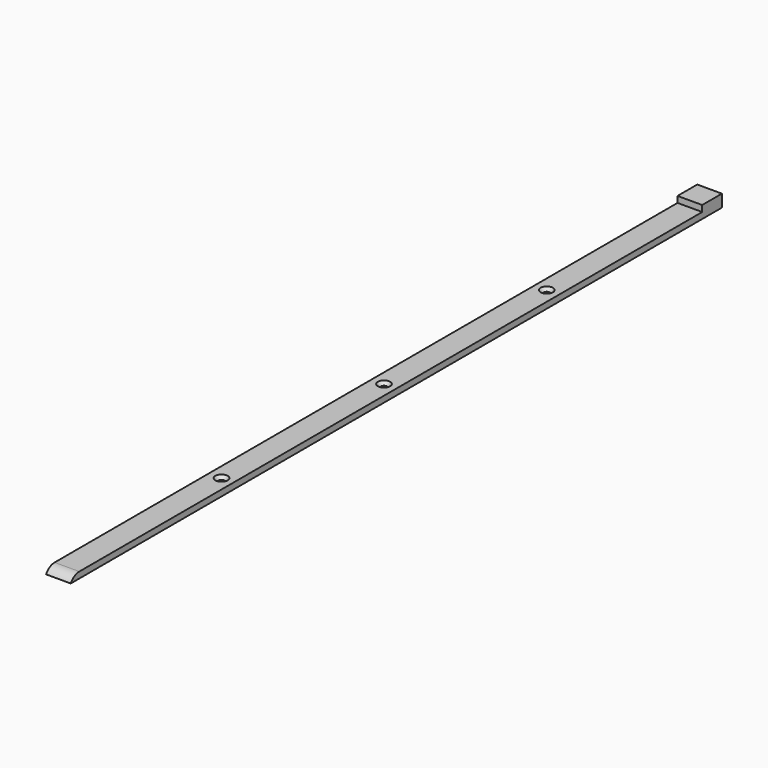
from build123d import *

# Parameters (mm, degrees)
F0_W           = 10
F0_H           = 320
F1_DEPTH       = 2.5
F0_H_2         = 10
F2_DEPTH       = 5
F3_T1_DEPTH    = 31.6506350946
F5_D           = 2.5
F5_DEPTH       = 2.5
F5_CSINK_D     = 5
F5_CSINK_ANGLE = 90
F5_TIP         = 0.7510757738


# Not quite as in the source:
# - a fillet or chamfer that OpenCascade refuses, or shapes differently, is made with other operations: its cross-section is extruded or revolved along the edge and cut away or added


with BuildPart() as f1:
    # F0 (on Top) → F1 (new body)
    with BuildSketch(Plane.XY):
        with Locations((0, -5)):
            Rectangle(F0_W, F0_H)
    extrude(amount=F1_DEPTH)

    # F0 (on Top) → F2 (join)
    with BuildSketch(Plane.XY):
        with Locations((0, 160)):
            Rectangle(F0_W, F0_H_2)
    extrude(amount=F2_DEPTH)

    # F3: fillet of radius 5 on 1 edges, made by hand

    # F3_s2 → F3_t1 (cut)
    with BuildSketch(Plane.YZ.offset(-15.8253175473)):
        with BuildLine():
            ThreePointArc((-160.6698729811, 2.5), (-163.1698729811, 1.8301270189), (-165, 0))
            Line((-165, 0), (-165, 2.5))
            Line((-165, 2.5), (-160.6698729811, 2.5))
        make_face()
    extrude(amount=F3_T1_DEPTH, mode=Mode.SUBTRACT)

    # F5
    with Locations(Plane.XY.offset(2.5)):
        with Locations((0, 82.5), (0, 0), (0.1304344232, -82.5)):
            CounterSinkHole(F5_D / 2, F5_CSINK_D / 2, depth=F5_DEPTH, counter_sink_angle=F5_CSINK_ANGLE)
            with Locations((0, 0, -(F5_DEPTH + F5_TIP / 2))):  # 118° drill point
                Cone(0, F5_D / 2, F5_TIP, mode=Mode.SUBTRACT)


solid = f1.part
